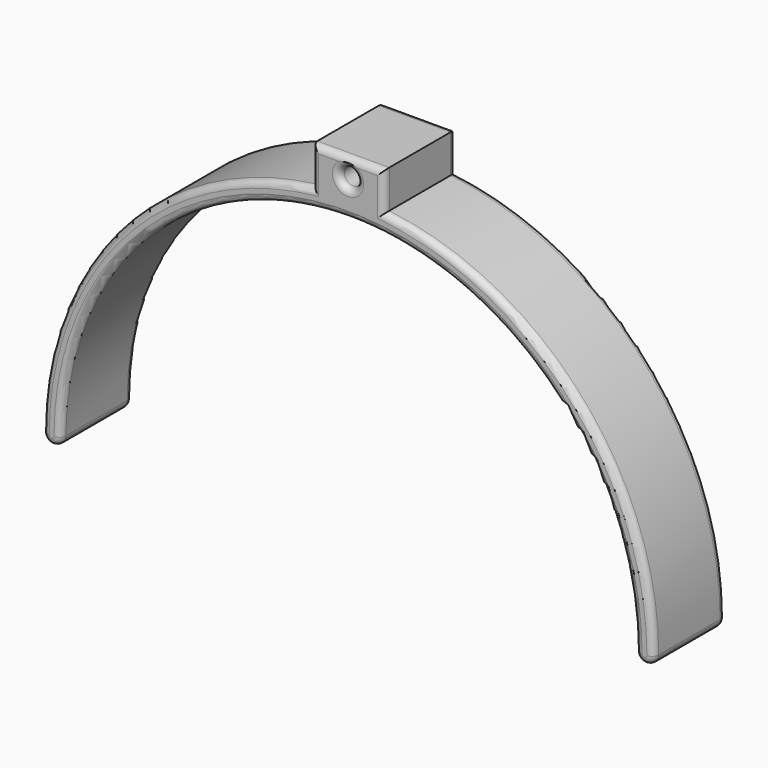
from build123d import *

# Parameters (mm, degrees)
F0_R          = 2.5
F1_DEPTH      = 25
F2_T3_ANGLE   = 180
F2_T6_ANGLE   = 180
F2_T9_ANGLE   = 180
F2_T12_ANGLE  = 86.3448287996
F2_T16_DEPTH  = 19.788438592
F2_S17_R      = 85
F2_T18_DEPTH  = 11
F2_T21_DEPTH  = 29.1981536726
F2_T24_DEPTH  = 19.788438592
F2_S25_R      = 85
F2_T26_DEPTH  = 11
F2_T29_ANGLE  = 86.3448287996
F2_T36_ANGLE  = 180
F2_T39_ANGLE  = 180
F2_T42_ANGLE  = 180
F2_T45_ANGLE  = 86.3448287996
F2_T49_DEPTH  = 19.788438592
F2_S50_R      = 85
F2_T51_DEPTH  = 11
F2_T54_DEPTH  = 29.1981536726
F2_T57_DEPTH  = 19.788438592
F2_S58_R      = 85
F2_T59_DEPTH  = 11
F2_T62_ANGLE  = 86.3448287996
F2_T70_ANGLE  = 86.3448287996
F2_T74_DEPTH  = 19.788438592
F2_S75_R      = 85
F2_T76_DEPTH  = 11
F2_T81_DEPTH  = 19.788438592
F2_S82_R      = 85
F2_T83_DEPTH  = 11
F2_T86_ANGLE  = 86.3448287996
F2_T92_DEPTH  = 19.788438592
F2_S93_R      = 85
F2_T94_DEPTH  = 11
F2_T97_ANGLE  = 86.3448287996
F2_T103_DEPTH = 19.788438592
F2_S104_R     = 85
F2_T105_DEPTH = 11
F2_T108_ANGLE = 86.3448287996


# Not quite as in the source:
# - a fillet or chamfer that OpenCascade refuses, or shapes differently, is made with other operations: its cross-section is extruded or revolved along the edge and cut away or added


with BuildPart() as f1:
    # F0 (on Front) → F1 (new body)
    with BuildSketch(Plane.XZ):
        with BuildLine():
            ThreePointArc((-80, 0), (0, 80), (80, 0))
            ThreePointArc((80, 0), (82.5, -2.5), (85, 0))
            ThreePointArc((85, 0), (63.5413251357, 56.4579489532), (10, 84.4097150807))
            Line((10, 84.4097150807), (10, 95))
            Line((10, 95), (0, 95))
            Line((0, 95), (-10, 95))
            Line((-10, 95), (-10, 84.4097150807))
            ThreePointArc((-10, 84.4097150807), (-63.5413251357, 56.4579489532), (-85, 0))
            ThreePointArc((-85, 0), (-82.5, -2.5), (-80, 0))
        make_face()
        with Locations((0, 89.7048575403)):
            Circle(F0_R, mode=Mode.SUBTRACT)
    extrude(amount=F1_DEPTH)

    # F2: fillet of radius 1.8396307345 on 18 edges, made by hand


with BuildPart() as f2_tool1:
    # F2_s2 → F2_t3 (revolve)
    with BuildSketch(Plane.XY):
        with BuildLine():
            ThreePointArc((-85, -23.1603692655), (-84.4611846327, -24.4611846327), (-83.1603692655, -25))
            Line((-83.1603692655, -25), (-85, -25))
            Line((-85, -25), (-85, -23.1603692655))
        make_face()
    revolve(axis=Axis((-82.5, -25, 0), (0, -1, 0)), revolution_arc=F2_T3_ANGLE)


with BuildPart() as f2_tool4:
    # F2_s5 → F2_t6 (revolve)
    with BuildSketch(Plane.XY):
        with BuildLine():
            ThreePointArc((-81.8396307345, -25), (-80.5388153673, -24.4611846327), (-80, -23.1603692655))
            Line((-80, -23.1603692655), (-80, -25))
            Line((-80, -25), (-81.8396307345, -25))
        make_face()
    revolve(axis=Axis((0, -25, 0), (0, 1, 0)), revolution_arc=F2_T6_ANGLE)


with BuildPart() as f2_tool7:
    # F2_s8 → F2_t9 (revolve)
    with BuildSketch(Plane.XY):
        with BuildLine():
            ThreePointArc((81.8396307345, -25), (80.5388153673, -24.4611846327), (80, -23.1603692655))
            Line((80, -23.1603692655), (80, -25))
            Line((80, -25), (81.8396307345, -25))
        make_face()
    revolve(axis=Axis((82.5, -25, 0), (0, -1, 0)), revolution_arc=F2_T9_ANGLE)


with BuildPart() as f2_tool10:
    # F2_s11 → F2_t12 (revolve)
    with BuildSketch(Plane.XY):
        with BuildLine():
            ThreePointArc((83.1603692655, -25), (84.4611846327, -24.4611846327), (85, -23.1603692655))
            Line((85, -23.1603692655), (85, -25))
            Line((85, -25), (83.1603692655, -25))
        make_face()
    revolve(axis=Axis((0, -25, 0), (0, -1, 0)), revolution_arc=F2_T12_ANGLE)

    split(bisect_by=Plane.YZ.offset(10), keep=Keep.TOP)


with BuildPart() as f2_tool14:
    # F2_s15 → F2_t16 (new body)
    with BuildSketch(Plane.XY.offset(79.8106382443)):
        with BuildLine():
            ThreePointArc((8.1603692655, -25), (9.4611846327, -24.4611846327), (10, -23.1603692655))
            Line((10, -23.1603692655), (10, -25))
            Line((10, -25), (8.1603692655, -25))
        make_face()
    extrude(amount=F2_T16_DEPTH)

    # F2_s17 → F2_t18 (cut, symmetric)
    with BuildSketch(Plane.XZ.offset(24.1)):
        Circle(F2_S17_R)
    extrude(amount=F2_T18_DEPTH, both=True, mode=Mode.SUBTRACT)


with BuildPart() as f2_tool19:
    # F2_s20 → F2_t21 (new body)
    with BuildSketch(Plane.YZ.offset(-14.5990768363)):
        with BuildLine():
            ThreePointArc((-25, 93.1603692655), (-24.4611846327, 94.4611846327), (-23.1603692655, 95))
            Line((-23.1603692655, 95), (-25, 95))
            Line((-25, 95), (-25, 93.1603692655))
        make_face()
    extrude(amount=F2_T21_DEPTH)


with BuildPart() as f2_tool22:
    # F2_s23 → F2_t24 (new body)
    with BuildSketch(Plane.XY.offset(99.5990768363)):
        with BuildLine():
            ThreePointArc((-8.1603692655, -25), (-9.4611846327, -24.4611846327), (-10, -23.1603692655))
            Line((-10, -23.1603692655), (-10, -25))
            Line((-10, -25), (-8.1603692655, -25))
        make_face()
    extrude(amount=-F2_T24_DEPTH)

    # F2_s25 → F2_t26 (cut, symmetric)
    with BuildSketch(Plane.XZ.offset(24.1)):
        Circle(F2_S25_R)
    extrude(amount=F2_T26_DEPTH, both=True, mode=Mode.SUBTRACT)


with BuildPart() as f2_tool27:
    # F2_s28 → F2_t29 (revolve)
    with BuildSketch(Plane(origin=(0, 0, 0), x_dir=(0, 1, 0), z_dir=(0.9979658036, 0, 0.0637515093))):
        with BuildLine():
            ThreePointArc((-25, 83.1603692655), (-24.4611846327, 84.4611846327), (-23.1603692655, 85))
            Line((-23.1603692655, 85), (-25, 85))
            Line((-25, 85), (-25, 83.1603692655))
        make_face()
    revolve(axis=Axis((0, -25, 0), (0, -1, 0)), revolution_arc=F2_T29_ANGLE)

    split(bisect_by=Plane.YZ.offset(-10), keep=Keep.BOTTOM)


with BuildPart() as f2_tool31:
    # F2_s32 → F2_t33 (revolve)
    with BuildSketch(Plane.XY.offset(89.7048575403)):
        with BuildLine():
            ThreePointArc((4.3396307345, -25), (3.0388153673, -24.4611846327), (2.5, -23.1603692655))
            Line((2.5, -23.1603692655), (2.5, -25))
            Line((2.5, -25), (4.3396307345, -25))
        make_face()
    revolve(axis=Axis((0, -25, 89.7048575403), (0, -1, 0)))


with BuildPart() as f2_tool34:
    # F2_s35 → F2_t36 (revolve)
    with BuildSketch(Plane.XY):
        with BuildLine():
            ThreePointArc((-85, -1.8396307345), (-84.4611846327, -0.5388153673), (-83.1603692655, 0))
            Line((-83.1603692655, 0), (-85, 0))
            Line((-85, 0), (-85, -1.8396307345))
        make_face()
    revolve(axis=Axis((-82.5, 0, 0), (0, -1, 0)), revolution_arc=F2_T36_ANGLE)


with BuildPart() as f2_tool37:
    # F2_s38 → F2_t39 (revolve)
    with BuildSketch(Plane.XY):
        with BuildLine():
            ThreePointArc((-81.8396307345, 0), (-80.5388153673, -0.5388153673), (-80, -1.8396307345))
            Line((-80, -1.8396307345), (-80, 0))
            Line((-80, 0), (-81.8396307345, 0))
        make_face()
    revolve(axis=Axis((0, 0, 0), (0, 1, 0)), revolution_arc=F2_T39_ANGLE)


with BuildPart() as f2_tool40:
    # F2_s41 → F2_t42 (revolve)
    with BuildSketch(Plane.XY):
        with BuildLine():
            ThreePointArc((80, -1.8396307345), (80.5388153673, -0.5388153673), (81.8396307345, 0))
            Line((81.8396307345, 0), (80, 0))
            Line((80, 0), (80, -1.8396307345))
        make_face()
    revolve(axis=Axis((82.5, 0, 0), (0, -1, 0)), revolution_arc=F2_T42_ANGLE)


with BuildPart() as f2_tool43:
    # F2_s44 → F2_t45 (revolve)
    with BuildSketch(Plane.XY):
        with BuildLine():
            ThreePointArc((85, -1.8396307345), (84.4611846327, -0.5388153673), (83.1603692655, 0))
            Line((83.1603692655, 0), (85, 0))
            Line((85, 0), (85, -1.8396307345))
        make_face()
    revolve(axis=Axis((0, 0, 0), (0, -1, 0)), revolution_arc=F2_T45_ANGLE)

    split(bisect_by=Plane.YZ.offset(10), keep=Keep.TOP)


with BuildPart() as f2_tool47:
    # F2_s48 → F2_t49 (new body)
    with BuildSketch(Plane.XY.offset(79.8106382443)):
        with BuildLine():
            ThreePointArc((10, -1.8396307345), (9.4611846327, -0.5388153673), (8.1603692655, 0))
            Line((8.1603692655, 0), (10, 0))
            Line((10, 0), (10, -1.8396307345))
        make_face()
    extrude(amount=F2_T49_DEPTH)

    # F2_s50 → F2_t51 (cut, symmetric)
    with BuildSketch(Plane.XZ.offset(0.9)):
        Circle(F2_S50_R)
    extrude(amount=F2_T51_DEPTH, both=True, mode=Mode.SUBTRACT)


with BuildPart() as f2_tool52:
    # F2_s53 → F2_t54 (new body)
    with BuildSketch(Plane.YZ.offset(14.5990768363)):
        with BuildLine():
            ThreePointArc((-1.8396307345, 95), (-0.5388153673, 94.4611846327), (0, 93.1603692655))
            Line((0, 93.1603692655), (0, 95))
            Line((0, 95), (-1.8396307345, 95))
        make_face()
    extrude(amount=-F2_T54_DEPTH)


with BuildPart() as f2_tool55:
    # F2_s56 → F2_t57 (new body)
    with BuildSketch(Plane.XY.offset(99.5990768363)):
        with BuildLine():
            ThreePointArc((-10, -1.8396307345), (-9.4611846327, -0.5388153673), (-8.1603692655, 0))
            Line((-8.1603692655, 0), (-10, 0))
            Line((-10, 0), (-10, -1.8396307345))
        make_face()
    extrude(amount=-F2_T57_DEPTH)

    # F2_s58 → F2_t59 (cut, symmetric)
    with BuildSketch(Plane.XZ.offset(0.9)):
        Circle(F2_S58_R)
    extrude(amount=F2_T59_DEPTH, both=True, mode=Mode.SUBTRACT)


with BuildPart() as f2_tool60:
    # F2_s61 → F2_t62 (revolve)
    with BuildSketch(Plane(origin=(0, 0, 0), x_dir=(0, 1, 0), z_dir=(0.9979658036, 0, 0.0637515093))):
        with BuildLine():
            ThreePointArc((0, 83.1603692655), (-0.5388153673, 84.4611846327), (-1.8396307345, 85))
            Line((-1.8396307345, 85), (0, 85))
            Line((0, 85), (0, 83.1603692655))
        make_face()
    revolve(axis=Axis((0, 0, 0), (0, -1, 0)), revolution_arc=F2_T62_ANGLE)

    split(bisect_by=Plane.YZ.offset(-10), keep=Keep.BOTTOM)


with BuildPart() as f2_tool64:
    # F2_s65 → F2_t66 (revolve)
    with BuildSketch(Plane.XY.offset(89.7048575403)):
        with BuildLine():
            ThreePointArc((2.5, -1.8396307345), (3.0388153673, -0.5388153673), (4.3396307345, 0))
            Line((4.3396307345, 0), (2.5, 0))
            Line((2.5, 0), (2.5, -1.8396307345))
        make_face()
    revolve(axis=Axis((0, 0, 89.7048575403), (0, -1, 0)))


with BuildPart() as f2_tool68:
    # F2_s69 → F2_t70 (revolve)
    with BuildSketch(Plane.XY):
        with BuildLine():
            ThreePointArc((83.1603692655, -25), (84.4611846327, -24.4611846327), (85, -23.1603692655))
            Line((85, -23.1603692655), (85, -25))
            Line((85, -25), (83.1603692655, -25))
        make_face()
    revolve(axis=Axis((0, -25, 0), (0, -1, 0)), revolution_arc=F2_T70_ANGLE)

    split(bisect_by=Plane.YZ.offset(10), keep=Keep.BOTTOM)


with BuildPart() as f2_tool72:
    # F2_s73 → F2_t74 (new body)
    with BuildSketch(Plane.XY.offset(79.8106382443)):
        with BuildLine():
            ThreePointArc((8.1603692655, -25), (9.4611846327, -24.4611846327), (10, -23.1603692655))
            Line((10, -23.1603692655), (10, -25))
            Line((10, -25), (8.1603692655, -25))
        make_face()
    extrude(amount=F2_T74_DEPTH)

    # F2_s75 → F2_t76 (intersect, symmetric)
    with BuildSketch(Plane.XZ.offset(24.1)):
        Circle(F2_S75_R)
    extrude(amount=F2_T76_DEPTH, both=True, mode=Mode.INTERSECT)


with BuildPart() as f2_tool68_1:
    add(f2_tool68.part)

    # F2_t77: intersect F2_tool72
    add(f2_tool72.part, mode=Mode.INTERSECT)


with BuildPart() as f2_tool79:
    # F2_s80 → F2_t81 (new body)
    with BuildSketch(Plane.XY.offset(99.5990768363)):
        with BuildLine():
            ThreePointArc((-8.1603692655, -25), (-9.4611846327, -24.4611846327), (-10, -23.1603692655))
            Line((-10, -23.1603692655), (-10, -25))
            Line((-10, -25), (-8.1603692655, -25))
        make_face()
    extrude(amount=-F2_T81_DEPTH)

    # F2_s82 → F2_t83 (intersect, symmetric)
    with BuildSketch(Plane.XZ.offset(24.1)):
        Circle(F2_S82_R)
    extrude(amount=F2_T83_DEPTH, both=True, mode=Mode.INTERSECT)


with BuildPart() as f2_tool84:
    # F2_s85 → F2_t86 (revolve)
    with BuildSketch(Plane(origin=(0, 0, 0), x_dir=(0, 1, 0), z_dir=(0.9979658036, 0, 0.0637515093))):
        with BuildLine():
            ThreePointArc((-25, 83.1603692655), (-24.4611846327, 84.4611846327), (-23.1603692655, 85))
            Line((-23.1603692655, 85), (-25, 85))
            Line((-25, 85), (-25, 83.1603692655))
        make_face()
    revolve(axis=Axis((0, -25, 0), (0, -1, 0)), revolution_arc=F2_T86_ANGLE)

    split(bisect_by=Plane.YZ.offset(-10), keep=Keep.TOP)


with BuildPart() as f2_tool79_1:
    add(f2_tool79.part)

    # F2_t88: intersect F2_tool84
    add(f2_tool84.part, mode=Mode.INTERSECT)


with BuildPart() as f2_tool90:
    # F2_s91 → F2_t92 (new body)
    with BuildSketch(Plane.XY.offset(79.8106382443)):
        with BuildLine():
            ThreePointArc((10, -1.8396307345), (9.4611846327, -0.5388153673), (8.1603692655, 0))
            Line((8.1603692655, 0), (10, 0))
            Line((10, 0), (10, -1.8396307345))
        make_face()
    extrude(amount=F2_T92_DEPTH)

    # F2_s93 → F2_t94 (intersect, symmetric)
    with BuildSketch(Plane.XZ.offset(0.9)):
        Circle(F2_S93_R)
    extrude(amount=F2_T94_DEPTH, both=True, mode=Mode.INTERSECT)


with BuildPart() as f2_tool95:
    # F2_s96 → F2_t97 (revolve)
    with BuildSketch(Plane.XY):
        with BuildLine():
            ThreePointArc((85, -1.8396307345), (84.4611846327, -0.5388153673), (83.1603692655, 0))
            Line((83.1603692655, 0), (85, 0))
            Line((85, 0), (85, -1.8396307345))
        make_face()
    revolve(axis=Axis((0, 0, 0), (0, -1, 0)), revolution_arc=F2_T97_ANGLE)

    split(bisect_by=Plane.YZ.offset(10), keep=Keep.BOTTOM)


with BuildPart() as f2_tool90_1:
    add(f2_tool90.part)

    # F2_t99: intersect F2_tool95
    add(f2_tool95.part, mode=Mode.INTERSECT)


with BuildPart() as f2_tool101:
    # F2_s102 → F2_t103 (new body)
    with BuildSketch(Plane.XY.offset(99.5990768363)):
        with BuildLine():
            ThreePointArc((-10, -1.8396307345), (-9.4611846327, -0.5388153673), (-8.1603692655, 0))
            Line((-8.1603692655, 0), (-10, 0))
            Line((-10, 0), (-10, -1.8396307345))
        make_face()
    extrude(amount=-F2_T103_DEPTH)

    # F2_s104 → F2_t105 (intersect, symmetric)
    with BuildSketch(Plane.XZ.offset(0.9)):
        Circle(F2_S104_R)
    extrude(amount=F2_T105_DEPTH, both=True, mode=Mode.INTERSECT)


with BuildPart() as f2_tool106:
    # F2_s107 → F2_t108 (revolve)
    with BuildSketch(Plane(origin=(0, 0, 0), x_dir=(0, 1, 0), z_dir=(0.9979658036, 0, 0.0637515093))):
        with BuildLine():
            ThreePointArc((0, 83.1603692655), (-0.5388153673, 84.4611846327), (-1.8396307345, 85))
            Line((-1.8396307345, 85), (0, 85))
            Line((0, 85), (0, 83.1603692655))
        make_face()
    revolve(axis=Axis((0, 0, 0), (0, -1, 0)), revolution_arc=F2_T108_ANGLE)

    split(bisect_by=Plane.YZ.offset(-10), keep=Keep.TOP)


with BuildPart() as f2_tool101_1:
    add(f2_tool101.part)

    # F2_t110: intersect F2_tool106
    add(f2_tool106.part, mode=Mode.INTERSECT)


with BuildPart() as f1_1:
    add(f1.part)

    # F2_t111: cut F2_tool1, F2_tool4, F2_tool7, F2_tool10, F2_tool14, F2_tool19, F2_tool22, F2_tool27, F2_tool31, F2_tool34, F2_tool37, F2_tool40, F2_tool43, F2_tool47, F2_tool52, F2_tool55, F2_tool60, F2_tool64, F2_tool68, F2_tool79, F2_tool90, F2_tool101
    add([f2_tool1.part, f2_tool4.part, f2_tool7.part, f2_tool10.part, f2_tool14.part, f2_tool19.part, f2_tool22.part, f2_tool27.part, f2_tool31.part, f2_tool34.part, f2_tool37.part, f2_tool40.part, f2_tool43.part, f2_tool47.part, f2_tool52.part, f2_tool55.part, f2_tool60.part, f2_tool64.part, f2_tool68_1.part, f2_tool79_1.part, f2_tool90_1.part, f2_tool101_1.part], mode=Mode.SUBTRACT)


solid = f1_1.part
